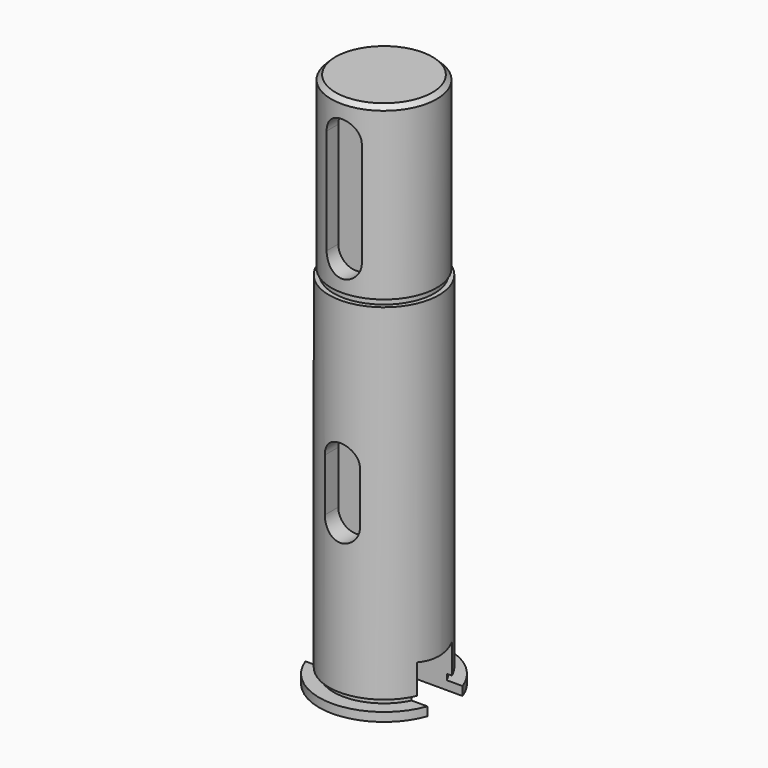
from build123d import *

# Parameters (mm, degrees)
F2_R          = 30
F3_DEPTH      = 5
F3_DEPTH_BACK = 5
F6_DEPTH      = 25
F8_DEPTH      = 25
F9_SIZE       = 1


# Not quite as in the source:
# - a pattern or mirror of a feature is missing from the dataset's text; its kind, count and spacing are read off the source's solid


with BuildPart() as f1:
    # F0 (on Front) → F1 (revolve)
    with BuildSketch(Plane.XZ):
        Polygon((-14.75, -2), (0, -2), (0, 120), (-12, 120), (-12, 81.2), (-11.45, 81.2), (-11.45, 79.9), (-12.5, 79.9), (-12.5, 1.3), (-11.45, 1.3), (-11.45, 0), (-14.75, 0), align=None)
    revolve(axis=Axis((0, 0, 59), (0, 0, -1)))

    # F2 (on Front) → F3 (cut, two sides)
    with BuildSketch(Plane.XZ) as f3_sk:
        with Locations((0, -19.7)):
            Circle(F2_R)
    extrude(amount=-F3_DEPTH, mode=Mode.SUBTRACT)
    extrude(f3_sk.sketch, amount=F3_DEPTH_BACK, mode=Mode.SUBTRACT)

    # F5 (on offset) → F6 (cut)
    with BuildSketch(Plane.XZ.offset(8)):
        with BuildLine():
            ThreePointArc((4, 112), (0, 116), (-4, 112))
            Line((-4, 112), (-4, 88))
            ThreePointArc((-4, 88), (0, 84), (4, 88))
            Line((4, 88), (4, 112))
        make_face()
    extrude(amount=F6_DEPTH, mode=Mode.SUBTRACT)

    # F7 (on offset) → F8 (cut)
    with BuildSketch(Plane.XZ.offset(8)):
        with BuildLine():
            ThreePointArc((4, 47.3), (0, 51.3), (-4, 47.3))
            Line((-4, 47.3), (-4, 35.3))
            ThreePointArc((-4, 35.3), (0, 31.3), (4, 35.3))
            Line((4, 35.3), (4, 47.3))
        make_face()
    f8 = extrude(amount=F8_DEPTH, mode=Mode.SUBTRACT)

    # F8_copies: F8 across plane
    add(f8.mirror(Plane.ZX), mode=Mode.SUBTRACT)

    # F9
    f9_edges = [f1.edges().sort_by_distance(p)[0] for p in [
        (12, 0, 120),
    ]]
    chamfer(f9_edges, length=F9_SIZE)


solid = f1.part
